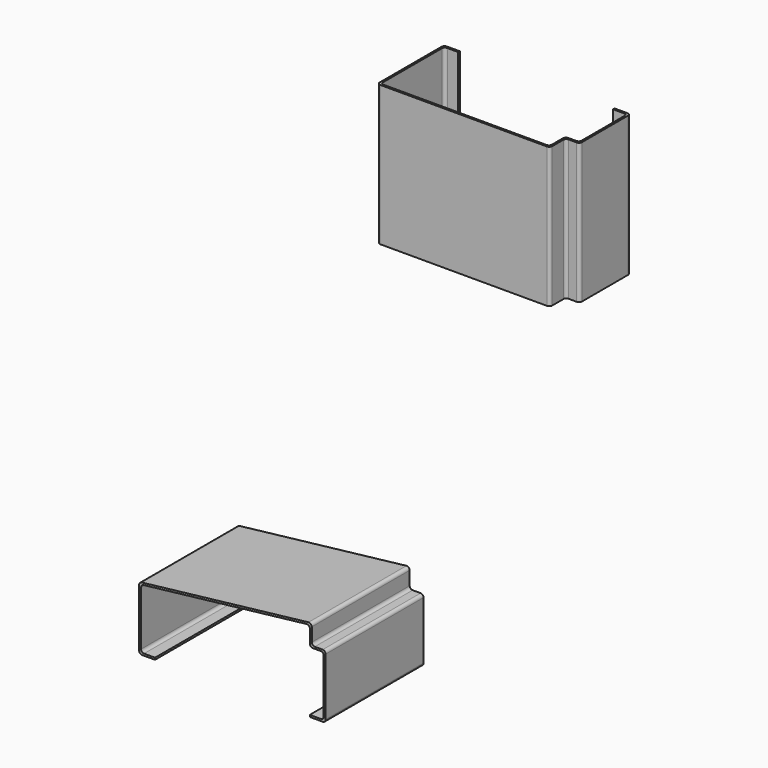
from build123d import *

# Parameters (mm, degrees)
F1_DEPTH       = 304.8
F3_DEPTH       = 254
F3_DEPTH_BACK  = 50.8
F6_DEPTH       = 15.875
F8_DEPTH       = 66.676
F11_W          = 2.1258684099
F11_H          = 0.0508
F12_DEPTH      = 254.001
F13_W          = 299.0930452943
F13_H          = 280.027359724
F14_DEPTH      = 74.6135
F14_DEPTH_BACK = 74.6135
F15_R          = 2.38125
F16_R          = 2.38125


# Not quite as in the source:
# - a feature of the source that left no trace in its solid (it failed there, or was rolled back) is left out


with BuildPart() as f1:
    # F0 (on Front) → F1 (new body)
    with BuildSketch(Plane.XZ):
        Polygon((-74.6125, -50.8), (-61.9125, -50.8), (-61.9125, -49.276), (-73.0885, -49.276), (-73.0885, -1.3588619322), (61.976, 14.1657932403), (61.976, -1.524), (73.0885, -1.524), (73.0885, -49.276), (61.9125, -49.276), (61.9125, -50.8), (74.6125, -50.8), (74.6125, 0), (63.5, 0), (63.5, 15.875), (-74.6125, 0), align=None)
    extrude(amount=-F1_DEPTH)


with BuildPart() as f3:
    # F2 (on Top) → F3 (new body, two sides)
    with BuildSketch(Plane.XY) as f3_sk:
        Polygon((-61.9125, 304.8), (-74.6125, 304.8), (-74.6125, 238.125), (63.5, 238.125), (63.5, 254), (74.6125, 254), (74.6125, 304.8), (61.976, 304.8), (61.976, 303.276), (73.0885, 303.276), (73.0885, 255.524), (61.976, 255.524), (61.976, 239.649), (-73.0885, 239.649), (-73.0885, 303.276), (-61.9125, 303.276), align=None)
    extrude(amount=F3_DEPTH)
    extrude(f3_sk.sketch, amount=-F3_DEPTH_BACK)


with BuildPart() as f6_tool:
    # F5 (on face) → F6 (new body, through all)
    with BuildSketch(Plane.XZ.offset(-238.125)):
        Polygon((61.976, 14.1657932403), (-73.0885, -1.3588619322), (-91.1419016793, -3.4339655735), (-91.1419016793, -71.0971727967), (86.3244011998, -71.0971727967), (86.3244011998, 0), (61.976, 0), align=None)
    extrude(amount=-F6_DEPTH)


with BuildPart() as f1_1:
    add(f1.part)

    # F6: cut by f6_tool
    add(f6_tool.part, mode=Mode.SUBTRACT)


with BuildPart() as f3_1:
    add(f3.part)

    # F6: cut by f6_tool
    add(f6_tool.part, mode=Mode.SUBTRACT)


with BuildPart() as f8_tool:
    # F7 (on face) → F8 (new body, through all)
    with BuildSketch(Plane.XZ.offset(-238.125)):
        Polygon((-74.6125, 0), (-74.6125, -1.5340343459), (61.976, 14.1657932403), (61.976, 0), (63.5, 0), (63.5, 15.875), align=None)
    extrude(amount=-F8_DEPTH)


with BuildPart() as f1_2:
    add(f1_1.part)

    # F8: cut by f8_tool
    add(f8_tool.part, mode=Mode.SUBTRACT)


with BuildPart() as f3_2:
    add(f3_1.part)

    # F8: cut by f8_tool
    add(f8_tool.part, mode=Mode.SUBTRACT)


with BuildPart() as f1_3:
    add(f1_2.part)

    # F10: union F3
    add(f3_2.part)

    # F11 (on face) → F12 (cut, through all)
    with BuildSketch(Plane.XY):
        with Locations((62.4370657951, 238.0996)):
            Rectangle(F11_W, F11_H)
    extrude(amount=F12_DEPTH, mode=Mode.SUBTRACT)

    # F13 (on Right) → F14 (cut, two sides)
    with BuildSketch(Plane.YZ) as f14_sk:
        with Locations((247.4853210151, 1.7642229795)):
            Rectangle(F13_W, F13_H)
    extrude(amount=-F14_DEPTH, mode=Mode.SUBTRACT)
    extrude(f14_sk.sketch, amount=F14_DEPTH_BACK, mode=Mode.SUBTRACT)

    # F15
    f15_edges = [f1_3.edges().sort_by_distance(p)[0] for p in [
        (-73.0885, 239.649, 197.888951),
        (-74.6125, 238.125, 197.888951),
        (-74.6125, 304.8, 197.888951),
        (-73.0885, 303.276, 197.888951),
        (61.976, 239.649, 197.888951),
        (61.976, 255.524, 197.888951),
        (73.0885, 255.524, 197.888951),
        (73.0885, 303.276, 197.888951),
        (63.5, 238.125, 197.888951),
        (63.5, 254, 197.888951),
        (74.6125, 254, 197.888951),
        (74.6125, 304.8, 197.888951),
    ]]
    fillet(f15_edges, radius=F15_R)

    # F16
    f16_edges = [f1_3.edges().sort_by_distance(p)[0] for p in [
        (-73.0885, 48.969399, -49.276),
        (-73.0885, 48.969399, -1.358862),
        (61.976, 48.969399, 14.165793),
        (61.976, 48.969399, -1.524),
        (73.0885, 48.969399, -1.524),
        (73.0885, 48.969399, -49.276),
        (74.6125, 48.969399, -50.8),
        (74.6125, 48.969399, 0),
        (63.5, 48.969399, 15.875),
        (-74.6125, 48.969399, 0),
        (-74.6125, 48.969399, -50.8),
        (63.5, 48.969399, 0),
    ]]
    fillet(f16_edges, radius=F16_R)


solid = f1_3.part
